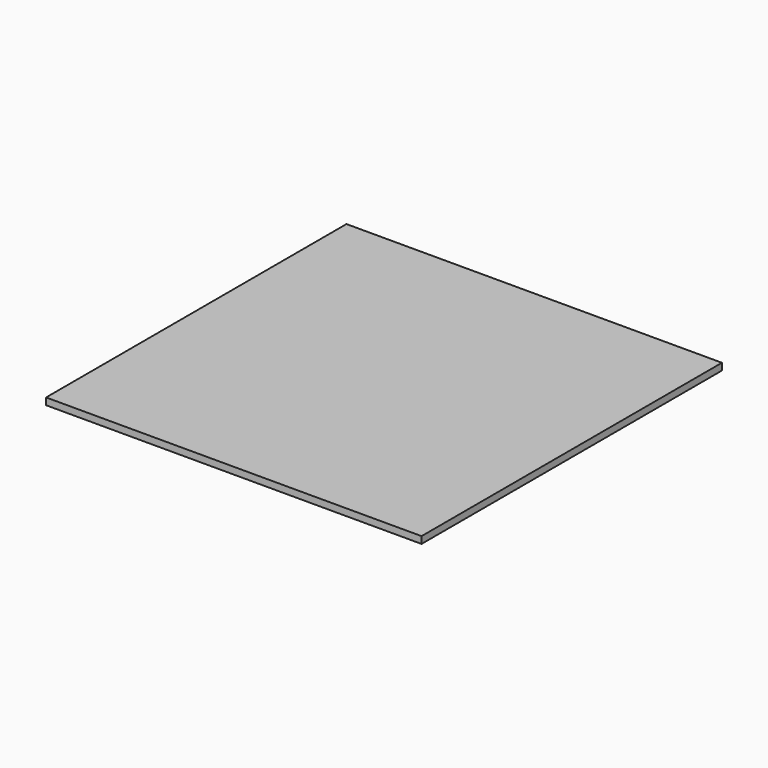
from build123d import *

# Parameters (mm, degrees)
F0_W     = 6
F0_H     = 6
F1_DEPTH = 0.06
F2_SCALE = 10
F5_START = -2
F4_W     = 60
F4_H     = 60
F5_DEPTH = 0.5
F6_SCALE = 0.903


# Not quite as in the source:
# - a feature names something its author has since deleted; it is built from what else it names


with BuildPart() as f1:
    # F0 (on Top) → F1 (new body)
    with BuildSketch(Plane.XY):
        Rectangle(F0_W, F0_H)
    extrude(amount=F1_DEPTH)


with BuildPart() as f1_1:
    # F2: moved
    add(f1.part.scale(F2_SCALE))

    # F4 (on offset) → F5 (join)
    with BuildSketch(Plane.XY.offset(2).offset(F5_START)):
        Rectangle(F4_W, F4_H)
    extrude(amount=-F5_DEPTH)


with BuildPart() as f1_2:
    # F6: moved
    add(f1_1.part.scale(F6_SCALE))


solid = f1_2.part
